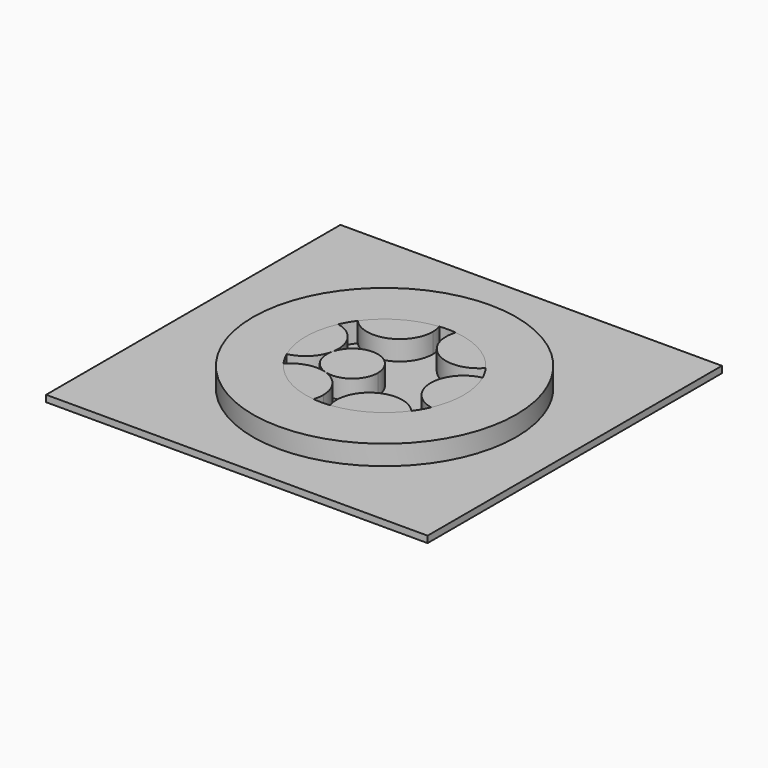
from build123d import *

# Parameters (mm, degrees)
F1_DEPTH = 0.3
F0_R     = 2
F2_DEPTH = 0.3
F3_DEPTH = 0.3
F5_W     = 5.7901758701
F5_H     = 5.5838446133
F6_DEPTH = 0.1


# Not quite as in the source:
# - a feature of the source that left no trace in its solid (it failed there, or was rolled back) is left out


with BuildPart() as f1:
    # F0 (on Top) → F1 (new body)
    with BuildSketch(Plane.XY):
        with BuildLine():
            ThreePointArc((-0.7096651668, -0.0978353275), (-0.7024221585, -0.04915579), (-0.7, 0))
            ThreePointArc((-0.7, 0), (-0.8113592061, 0.3145764348), (-1.0958333333, 0.4890289414))
            ThreePointArc((-1.0958333333, 0.4890289414), (-1.2, 0), (-1.0958333333, -0.4890289414))
            ThreePointArc((-1.0958333333, -0.4890289414), (-0.8523553963, -0.3593650366), (-0.7146924586, -0.1203187029))
            ThreePointArc((-0.7146924586, -0.1203187029), (-0.7123462626, -0.1090395733), (-0.7096651668, -0.0978353275))
        make_face()
        with BuildLine():
            ThreePointArc((-0.7146924586, -0.1203187029), (-0.7120492993, -0.1091059745), (-0.7096651668, -0.0978353275))
            ThreePointArc((-0.7096651668, -0.0978353275), (-0.7123462626, -0.1090395733), (-0.7146924586, -0.1203187029))
        make_face()
    extrude(amount=F1_DEPTH)


with BuildPart() as f1b:
    # F0 (on Top) → F1, piece 2 (new body)
    with BuildSketch(Plane.XY):
        with BuildLine():
            ThreePointArc((-0.1244051802, 1.1935339757), (-0.6, 1.0392304845), (-0.9714281531, 0.7045050343))
            ThreePointArc((-0.9714281531, 0.7045050343), (-0.420715417, 0.5724789036), (-0.1, 1.0392304845))
            ThreePointArc((-0.1, 1.0392304845), (-0.1061389822, 1.1173412716), (-0.1244051802, 1.1935339757))
        make_face()
    extrude(amount=F1_DEPTH)


with BuildPart() as f1c:
    # F0 (on Top) → F1, piece 3 (new body)
    with BuildSketch(Plane.XY):
        with BuildLine():
            ThreePointArc((-0.46298597, -0.5583696361), (-0.7381172832, -0.5586853607), (-0.9714281531, -0.7045050343))
            ThreePointArc((-0.9714281531, -0.7045050343), (-0.6, -1.0392304845), (-0.1244051802, -1.1935339757))
            ThreePointArc((-0.1244051802, -1.1935339757), (-0.1061389822, -1.1173412716), (-0.1, -1.0392304845))
            ThreePointArc((-0.1, -1.0392304845), (-0.1931954282, -0.748524378), (-0.4380401615, -0.5661881918))
            ThreePointArc((-0.4380401615, -0.5661881918), (-0.4505791453, -0.5624897467), (-0.46298597, -0.5583696361))
        make_face()
        with BuildLine():
            ThreePointArc((-0.4380401615, -0.5661881918), (-0.4504619581, -0.5621158505), (-0.46298597, -0.5583696361))
            ThreePointArc((-0.46298597, -0.5583696361), (-0.4505791453, -0.5624897467), (-0.4380401615, -0.5661881918))
        make_face()
    extrude(amount=F1_DEPTH)


with BuildPart() as f1d:
    # F0 (on Top) → F1, piece 4 (new body)
    with BuildSketch(Plane.XY):
        with BuildLine():
            ThreePointArc((1.1, 1.0392304845), (0.678110787, 1.5330915024), (0.1244051802, 1.1935339757))
            ThreePointArc((0.1244051802, 1.1935339757), (0.6, 1.0392304845), (0.9714281531, 0.7045050343))
            ThreePointArc((0.9714281531, 0.7045050343), (1.0667515809, 0.8599459015), (1.1, 1.0392304845))
        make_face()
    extrude(amount=F1_DEPTH)



with BuildPart() as f1e:
    # F0 (on Top) → F1, piece 5 (new body)
    with BuildSketch(Plane.XY):
        with BuildLine():
            ThreePointArc((0.9714281531, -0.7045050343), (0.6, -1.0392304845), (0.1244051802, -1.1935339757))
            ThreePointArc((0.1244051802, -1.1935339757), (0.678110787, -1.5330915024), (1.1, -1.0392304845))
            ThreePointArc((1.1, -1.0392304845), (1.0667515809, -0.8599459015), (0.9714281531, -0.7045050343))
        make_face()
    extrude(amount=F1_DEPTH)


with BuildPart() as f1f:
    # F0 (on Top) → F1, piece 6 (new body)
    with BuildSketch(Plane.XY):
        with BuildLine():
            ThreePointArc((1.2, 0), (1.1736694594, 0.25), (1.0958333333, 0.4890289414))
            ThreePointArc((1.0958333333, 0.4890289414), (0.7, 0), (1.0958333333, -0.4890289414))
            ThreePointArc((1.0958333333, -0.4890289414), (1.1736694594, -0.25), (1.2, 0))
        make_face()
    extrude(amount=F1_DEPTH)


with BuildPart() as f1d_1:
    add(f1d.part)

    add(f1e.part)  # F2 merges F1e
    # F0 (on Top) → F2 (join)
    with BuildSketch(Plane.XY):
        Circle(F0_R)
        with BuildLine():
            ThreePointArc((-1.0958333333, -0.4890289414), (-1.7, 0), (-1.0958333333, 0.4890289414))
            ThreePointArc((-1.0958333333, 0.4890289414), (-1.0392304845, 0.6), (-0.9714281531, 0.7045050343))
            ThreePointArc((-0.9714281531, 0.7045050343), (-0.85, 1.4722431864), (-0.1244051802, 1.1935339757))
            ThreePointArc((-0.1244051802, 1.1935339757), (0, 1.2), (0.1244051802, 1.1935339757))
            ThreePointArc((0.1244051802, 1.1935339757), (0.678110787, 1.5330915024), (1.1, 1.0392304845))
            ThreePointArc((1.1, 1.0392304845), (1.0667515809, 0.8599459015), (0.9714281531, 0.7045050343))
            ThreePointArc((0.9714281531, 0.7045050343), (1.0392304845, 0.6), (1.0958333333, 0.4890289414))
            ThreePointArc((1.0958333333, 0.4890289414), (1.5145764348, 0.3886407939), (1.7, 0))
            ThreePointArc((1.7, 0), (1.5145764348, -0.3886407939), (1.0958333333, -0.4890289414))
            ThreePointArc((1.0958333333, -0.4890289414), (1.0392304845, -0.6), (0.9714281531, -0.7045050343))
            ThreePointArc((0.9714281531, -0.7045050343), (1.0667515809, -0.8599459015), (1.1, -1.0392304845))
            ThreePointArc((1.1, -1.0392304845), (0.678110787, -1.5330915024), (0.1244051802, -1.1935339757))
            ThreePointArc((0.1244051802, -1.1935339757), (0, -1.2), (-0.1244051802, -1.1935339757))
            ThreePointArc((-0.1244051802, -1.1935339757), (-0.85, -1.4722431864), (-0.9714281531, -0.7045050343))
            ThreePointArc((-0.9714281531, -0.7045050343), (-1.0392304845, -0.6), (-1.0958333333, -0.4890289414))
        make_face(mode=Mode.SUBTRACT)
        with BuildLine():
            ThreePointArc((-1.0958333333, -0.4890289414), (-1.2, 0), (-1.0958333333, 0.4890289414))
            ThreePointArc((-1.0958333333, 0.4890289414), (-1.7, 0), (-1.0958333333, -0.4890289414))
        make_face()
        with BuildLine():
            ThreePointArc((-0.1244051802, -1.1935339757), (-0.6, -1.0392304845), (-0.9714281531, -0.7045050343))
            ThreePointArc((-0.9714281531, -0.7045050343), (-0.85, -1.4722431864), (-0.1244051802, -1.1935339757))
        make_face()
        with BuildLine():
            ThreePointArc((1.7, 0), (1.5145764348, 0.3886407939), (1.0958333333, 0.4890289414))
            ThreePointArc((1.0958333333, 0.4890289414), (1.1736694594, 0.25), (1.2, 0))
            ThreePointArc((1.2, 0), (1.1736694594, -0.25), (1.0958333333, -0.4890289414))
            ThreePointArc((1.0958333333, -0.4890289414), (1.5145764348, -0.3886407939), (1.7, 0))
        make_face()
        with BuildLine():
            ThreePointArc((-0.1244051802, 1.1935339757), (-0.85, 1.4722431864), (-0.9714281531, 0.7045050343))
            ThreePointArc((-0.9714281531, 0.7045050343), (-0.6, 1.0392304845), (-0.1244051802, 1.1935339757))
        make_face()
    extrude(amount=F2_DEPTH)


with BuildPart() as f2:
    # F0 (on Top) → F2, piece 2 (new body)
    with BuildSketch(Plane.XY):
        with BuildLine():
            ThreePointArc((0.9714281531, -0.7045050343), (0.35, -0.6062177826), (0.1244051802, -1.1935339757))
            ThreePointArc((0.1244051802, -1.1935339757), (0.6, -1.0392304845), (0.9714281531, -0.7045050343))
        make_face()
    extrude(amount=F2_DEPTH)


with BuildPart() as f2b:
    # F0 (on Top) → F2, piece 3 (new body)
    with BuildSketch(Plane.XY):
        with BuildLine():
            ThreePointArc((0.9714281531, 0.7045050343), (0.6, 1.0392304845), (0.1244051802, 1.1935339757))
            ThreePointArc((0.1244051802, 1.1935339757), (0.35, 0.6062177826), (0.9714281531, 0.7045050343))
        make_face()
    extrude(amount=F2_DEPTH)


with BuildPart() as f3:
    # F0 (on Top) → F3 (new body)
    with BuildSketch(Plane.XY):
        with BuildLine():
            ThreePointArc((0.0518479844, -0.1934346327), (-0.2867344533, 0.1903105649), (-0.7096651668, -0.0978353275))
            ThreePointArc((-0.7096651668, -0.0978353275), (-0.7120492993, -0.1091059745), (-0.7146924586, -0.1203187029))
            ThreePointArc((-0.7146924586, -0.1203187029), (-0.6702487628, -0.3861225462), (-0.46298597, -0.5583696361))
            ThreePointArc((-0.46298597, -0.5583696361), (-0.4504619581, -0.5621158505), (-0.4380401615, -0.5661881918))
            ThreePointArc((-0.4380401615, -0.5661881918), (-0.1007143125, -0.5012233635), (0.0518479844, -0.1934346327))
        make_face()
    extrude(amount=F3_DEPTH)


with BuildPart() as f6:
    # F5 (on face) → F6 (new body)
    with BuildSketch(Plane(origin=(0, 0, 0), x_dir=(1, 0, 0), z_dir=(0, 0, -1))):
        with Locations((-0.1344780903, -0.1563602127)):
            Rectangle(F5_W, F5_H)
    extrude(amount=F6_DEPTH)


solid = Compound([f1.part, f1b.part, f1c.part, f1f.part, f1d_1.part, f2.part, f2b.part, f3.part, f6.part])
